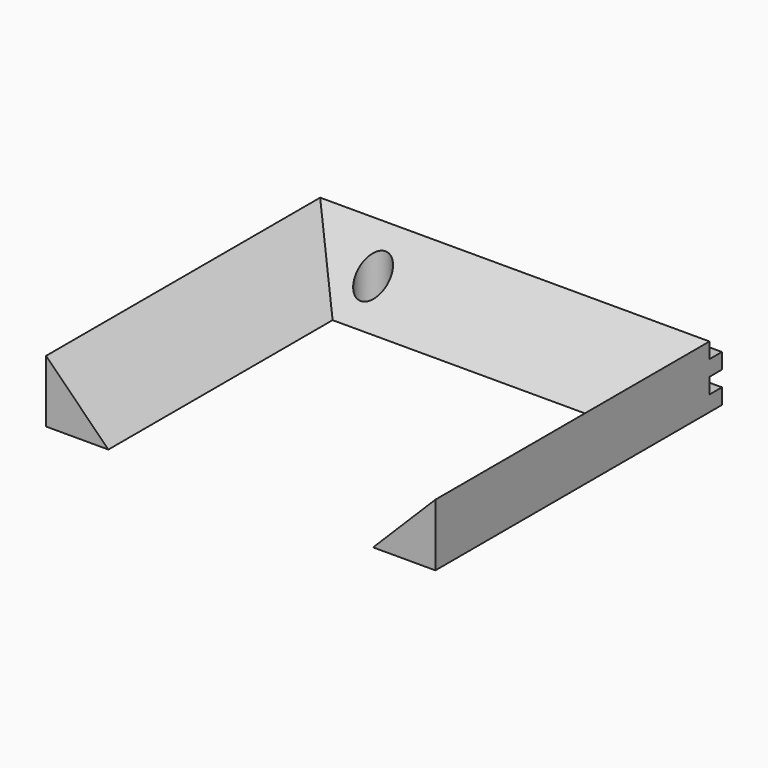
from build123d import *

# Parameters (mm, degrees)
F0_W     = 50.8
F0_H     = 228.6
F1_DEPTH = 50.8
F2_SIZE  = 50.79999
F4_R     = 12.7
F5_DEPTH = 63.5
F3_W     = 317.5
F3_H     = 12.7
F6_DEPTH = 12.7


# Not quite as in the source:
# - a fillet or chamfer is up to 0.001 mm smaller than in the source, because OpenCascade refuses the exact size


with BuildPart() as f1:
    # F0 (on Top) → F1 (new body)
    with BuildSketch(Plane.XY):
        with Locations((25.4, -114.3)):
            Rectangle(F0_W, F0_H)
        Polygon((0, 50.8), (0, 0), (50.8, 0), (266.7, 0), (317.5, 0), (317.5, 50.8), align=None)
        with Locations((292.1, -114.3)):
            Rectangle(F0_W, F0_H)
    extrude(amount=F1_DEPTH)

    # F2 (size 50.8 in the source; OpenCascade refuses exactly that, so slightly less here)
    f2_edges = [f1.edges().sort_by_distance(p)[0] for p in [
        (50.8, -114.3, 50.8),
        (158.75, 0, 50.8),
        (266.7, -114.3, 50.8),
    ]]
    chamfer(f2_edges, length=F2_SIZE)

    # F4 (on face) → F5 (cut)
    with BuildSketch(Plane(origin=(0, 0, 0), x_dir=(1, 0, 0), z_dir=(0, 0, -1))):
        with Locations((63.5, -25.4)):
            Circle(F4_R)
    extrude(amount=-F5_DEPTH, mode=Mode.SUBTRACT)

    # F3 (on face) → F6 (join)
    with BuildSketch(Plane(origin=(0, 50.8, 0), x_dir=(-1, 0, 0), z_dir=(0, 1, 0))):
        with Locations((-158.75, 6.35)):
            Rectangle(F3_W, F3_H)
        with Locations((-158.75, 31.75)):
            Rectangle(F3_W, F3_H)
    extrude(amount=F6_DEPTH)


solid = f1.part
